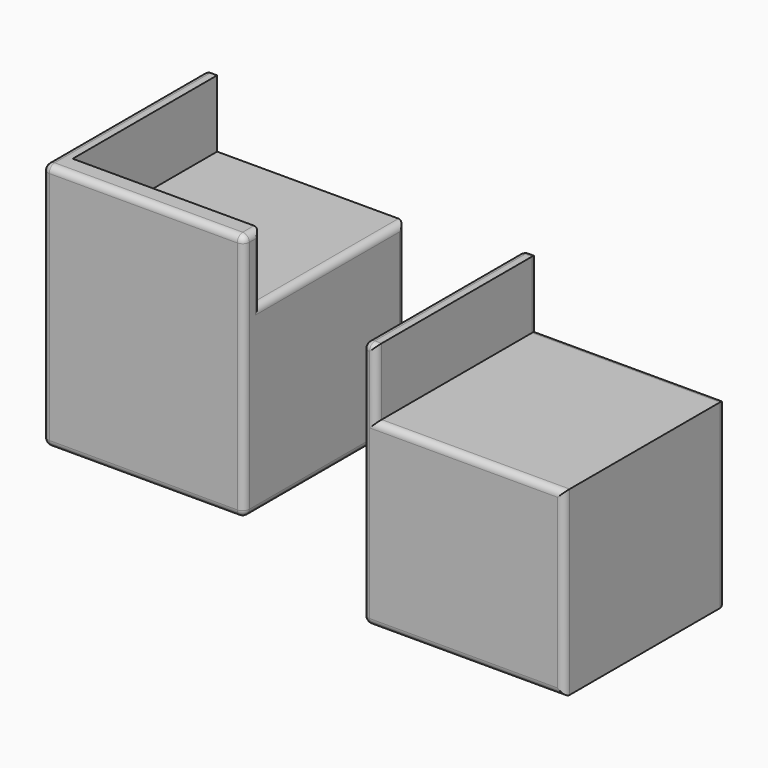
from build123d import *

# Parameters (mm, degrees)
F0_W     = 15
F0_H     = 15
F1_DEPTH = 13.5
F2_W     = 1
F2_H     = 13.4452538192
F2_H_2   = 1.5547461808
F2_W_2   = 14
F3_DEPTH = 5
F4_DEPTH = 5
F5_R     = 0.5
F6_W     = 15
F6_H     = 15
F7_DEPTH = 13.5
F8_W     = 1
F8_H     = 15
F9_DEPTH = 5
F10_R    = 0.49999


# Not quite as in the source:
# - a fillet or chamfer is up to 0.001 mm smaller than in the source, because OpenCascade refuses the exact size


with BuildPart() as f1:
    # F0 (on Top) → F1 (new body)
    with BuildSketch(Plane.XY):
        with Locations((-14.6885017678, -30.1897267997)):
            Rectangle(F0_W, F0_H)
    extrude(amount=F1_DEPTH)

    # F2 (on face) → F3 (join)
    with BuildSketch(Plane.XY.offset(13.5)):
        with Locations((-21.6885017678, -29.4123537093)):
            Rectangle(F2_W, F2_H)
        with Locations((-21.6885017678, -36.9123537093)):
            Rectangle(F2_W, F2_H_2)
        with Locations((-14.1885017678, -36.9123537093)):
            Rectangle(F2_W_2, F2_H_2)
    extrude(amount=F3_DEPTH)

    # F2 (on face) → F4 (join)
    with BuildSketch(Plane.XY.offset(13.5)):
        with Locations((-21.6885017678, -29.4123537093)):
            Rectangle(F2_W, F2_H)
        with Locations((-21.6885017678, -36.9123537093)):
            Rectangle(F2_W, F2_H_2)
        with Locations((-14.1885017678, -36.9123537093)):
            Rectangle(F2_W_2, F2_H_2)
    extrude(amount=F4_DEPTH)

    # F5
    f5_edges = [f1.edges().sort_by_distance(p)[0] for p in [
        (-22.188502, -30.189727, 18.5),
        (-22.188502, -37.689727, 9.25),
        (-22.188502, -30.189727, 0),
        (-22.188502, -22.689727, 9.25),
        (-14.688502, -37.689727, 18.5),
        (-7.188502, -37.689727, 9.25),
        (-14.688502, -37.689727, 0),
        (-7.188502, -30.189727, 0),
        (-14.688502, -22.689727, 0),
        (-7.188502, -36.912354, 18.5),
        (-7.188502, -36.134981, 16),
        (-7.188502, -29.412354, 13.5),
        (-7.188502, -22.689727, 6.75),
    ]]
    fillet(f5_edges, radius=F5_R)


with BuildPart() as f7:
    # F6 (on Top) → F7 (new body)
    with BuildSketch(Plane.XY):
        with Locations((13.8696695864, -36.0683391988)):
            Rectangle(F6_W, F6_H)
    extrude(amount=F7_DEPTH)

    # F8 (on face) → F9 (join)
    with BuildSketch(Plane.XY.offset(13.5)):
        with Locations((6.8696695864, -36.0683391988)):
            Rectangle(F8_W, F8_H)
    extrude(amount=F9_DEPTH)

    # F10 (radius 0.5 in the source; OpenCascade refuses exactly that, so slightly less here)
    f10_edges = [f7.edges().sort_by_distance(p)[0] for p in [
        (6.36967, -28.568339, 9.25),
        (6.36967, -36.068339, 18.5),
        (6.36967, -43.568339, 9.25),
        (6.36967, -36.068339, 0),
        (6.86967, -43.568339, 18.5),
        (7.36967, -43.568339, 16),
        (14.36967, -43.568339, 13.5),
        (21.36967, -43.568339, 6.75),
        (13.86967, -43.568339, 0),
        (21.36967, -28.568339, 6.75),
        (14.36967, -28.568339, 13.5),
        (7.36967, -28.568339, 16),
        (6.86967, -28.568339, 18.5),
        (13.86967, -28.568339, 0),
    ]]
    fillet(f10_edges, radius=F10_R)


solid = Compound([f1.part, f7.part])
